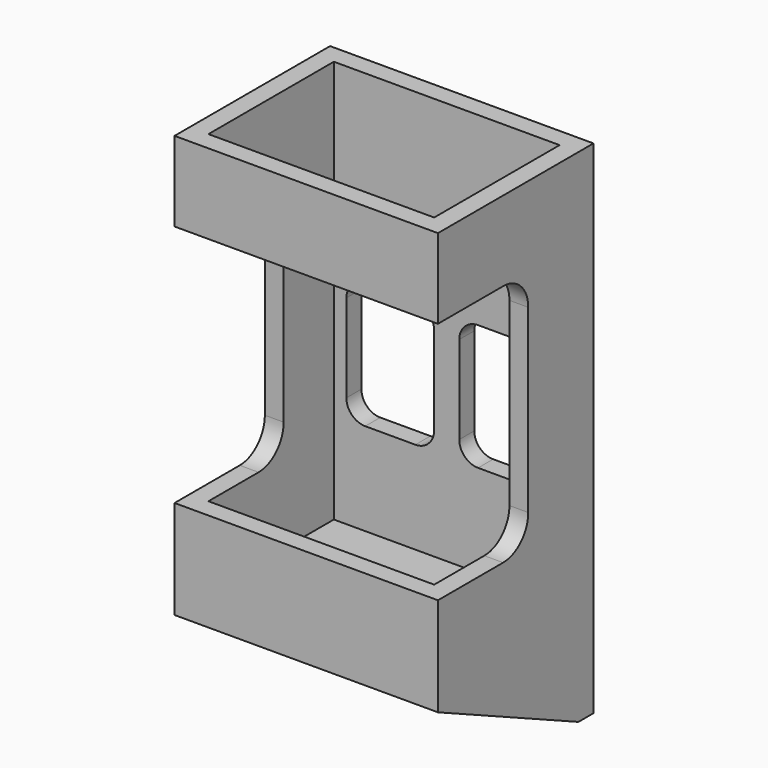
from build123d import *

# Parameters (mm, degrees)
F0_W      = 36
F0_H      = 12.73
F0_W_2    = 3
F1_DEPTH  = 31
F0_H_2    = 38.81
F2_DEPTH  = 13
F0_R      = 2.25
F3_DEPTH  = 3
F4_DEPTH  = 3
F5_DEPTH  = 31
F7_DEPTH  = 12.73
F8_W      = 36
F8_H      = 25
F9_DEPTH  = 25
F11_DEPTH = 25
F13_DEPTH = 25
F14_R     = 3.25
F14_R_2   = 2.25
F15_DEPTH = 1.5
F16_W     = 14
F16_H     = 20.04
F17_DEPTH = 25
F18_R     = 3
F19_R     = 5


# Not quite as in the source:
# - a feature names something its author has since deleted; it is built from what else it names


with BuildPart() as f1:
    # F0 (on Front) → F1 (new body)
    with BuildSketch(Plane.XZ):
        with Locations((21, 73.635)):
            Rectangle(F0_W, F0_H)
        with Locations((1.5, 73.635)):
            Rectangle(F0_W_2, F0_H)
        with Locations((40.5, 73.635)):
            Rectangle(F0_W_2, F0_H)
    extrude(amount=F1_DEPTH)



with BuildPart() as f1b:
    # F0 (on Front) → F1, piece 2 (new body)
    with BuildSketch(Plane.XZ):
        with Locations((40.5, 22.095)):
            Rectangle(F0_W_2, F0_H)
        with Locations((21, 22.095)):
            Rectangle(F0_W, F0_H)
        with Locations((1.5, 22.095)):
            Rectangle(F0_W_2, F0_H)
        Polygon((0, 15.73), (0, 12.73), (3, 12.73), (39, 12.73), (42, 12.73), (42, 15.73), (39, 15.73), (3, 15.73), align=None)
    extrude(amount=F1_DEPTH)


with BuildPart() as f1_1:
    add(f1.part)

    add(f1b.part)  # F2 merges F1b
    # F0 (on Front) → F2 (join)
    with BuildSketch(Plane.XZ):
        with Locations((40.5, 47.865)):
            Rectangle(F0_W_2, F0_H_2)
        with Locations((1.5, 47.865)):
            Rectangle(F0_W_2, F0_H_2)
    extrude(amount=F2_DEPTH)

    # F0 (on Front) → F3 (join)
    with BuildSketch(Plane.XZ):
        with Locations((21, 6.365)):
            Rectangle(F0_W, F0_H)
        with Locations((8.27, 6.37)):
            Circle(F0_R, mode=Mode.SUBTRACT)
        with Locations((21, 6.37)):
            Circle(F0_R, mode=Mode.SUBTRACT)
        with Locations((33.73, 6.37)):
            Circle(F0_R, mode=Mode.SUBTRACT)
    extrude(amount=F3_DEPTH)

    # F0 (on Front) → F4 (join)
    with BuildSketch(Plane.XZ):
        with Locations((21, 47.865)):
            Rectangle(F0_W, F0_H_2)
        with Locations((8.27, 58.87)):
            Circle(F0_R, mode=Mode.SUBTRACT)
        with Locations((21, 58.87)):
            Circle(F0_R, mode=Mode.SUBTRACT)
        with Locations((33.73, 58.87)):
            Circle(F0_R, mode=Mode.SUBTRACT)
    extrude(amount=F4_DEPTH)

    # F0 (on Front) → F5 (join)
    with BuildSketch(Plane.XZ):
        with Locations((40.5, 6.365)):
            Rectangle(F0_W_2, F0_H)
        with Locations((1.5, 6.365)):
            Rectangle(F0_W_2, F0_H)
    extrude(amount=F5_DEPTH)

    # F6 (on face) → F7 (cut)
    with BuildSketch(Plane.XY.offset(28.46)):
        Polygon((39, -3), (3, -3), (3, -13), (3, -28), (39, -28), (39, -13), align=None)
    extrude(amount=-F7_DEPTH, mode=Mode.SUBTRACT)

    # F8 (on face) → F9 (cut)
    with BuildSketch(Plane.XY.offset(80)):
        with Locations((21, -15.5)):
            Rectangle(F8_W, F8_H)
    extrude(amount=-F9_DEPTH, mode=Mode.SUBTRACT)

    # F10 (on face) → F11 (cut)
    with BuildSketch(Plane.YZ.offset(3)):
        Polygon((-3, 0), (-31, 12.73), (-31, 0), align=None)
    extrude(amount=-F11_DEPTH, mode=Mode.SUBTRACT)

    # F12 (on face) → F13 (cut)
    with BuildSketch(Plane(origin=(39, 0, 0), x_dir=(0, -1, 0), z_dir=(-1, 0, 0))):
        Polygon((31, 0), (31, 12.73), (3, 0), align=None)
    extrude(amount=-F13_DEPTH, mode=Mode.SUBTRACT)

    # F14 (on face) → F15 (cut)
    with BuildSketch(Plane.XZ.offset(3)):
        with Locations((8.27, 58.87)):
            Circle(F14_R)
        with Locations((8.27, 58.87)):
            Circle(F14_R_2, mode=Mode.SUBTRACT)
        with Locations((21, 58.87)):
            Circle(F14_R)
        with Locations((21, 58.87)):
            Circle(F14_R_2, mode=Mode.SUBTRACT)
        with Locations((33.73, 58.87)):
            Circle(F14_R)
        with Locations((33.73, 58.87)):
            Circle(F14_R_2, mode=Mode.SUBTRACT)
    extrude(amount=-F15_DEPTH, mode=Mode.SUBTRACT)

    # F16 (on face) → F17 (cut)
    with BuildSketch(Plane.XZ.offset(3)):
        with Locations((12, 40.48)):
            Rectangle(F16_W, F16_H)
        with Locations((30, 40.48)):
            Rectangle(F16_W, F16_H)
    extrude(amount=-F17_DEPTH, mode=Mode.SUBTRACT)

    # F18
    f18_edges = [f1_1.edges().sort_by_distance(p)[0] for p in [
        (5, -1.5, 50.5),
        (5, -1.5, 30.46),
        (37, -1.5, 30.46),
        (23, -1.5, 30.46),
        (19, -1.5, 30.46),
        (19, -1.5, 50.5),
        (23, -1.5, 50.5),
        (37, -1.5, 50.5),
    ]]
    fillet(f18_edges, radius=F18_R)

    # F19
    f19_edges = [f1_1.edges().sort_by_distance(p)[0] for p in [
        (1.5, -13, 67.27),
        (40.5, -13, 67.27),
        (1.5, -13, 28.46),
        (40.5, -13, 28.46),
    ]]
    fillet(f19_edges, radius=F19_R)


solid = f1_1.part
